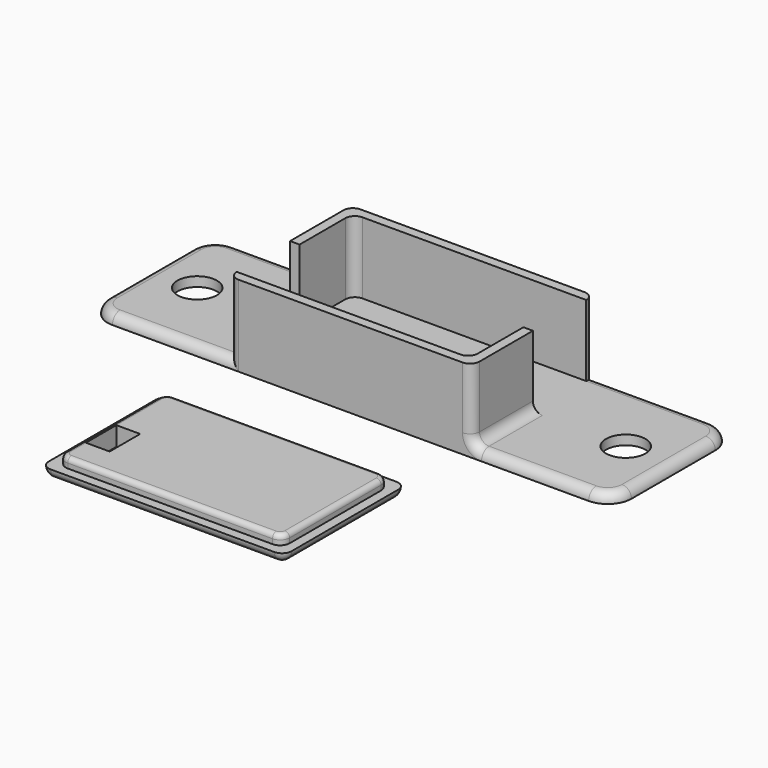
from build123d import *

# Parameters (mm, degrees)
F0_W      = 110
F0_H      = 32
F0_R      = 4.15
F1_DEPTH  = 2
F2_W      = 23.5
F2_H      = 2
F3_DEPTH  = 15
F4_W      = 14
F4_H      = 15
F5_DEPTH  = 2
F6_W      = 14
F6_H      = 15
F7_DEPTH  = 2
F8_R      = 5
F9_F1_R   = 2
F9_F2_R   = 1.9999
F10_W     = 51
F10_H     = 32
F10_W_2   = 47
F10_H_2   = 28
F11_DEPTH = 2
F12_W     = 23.5
F12_H     = 28
F13_DEPTH = 2
F14_R     = 1.99999
F15_R     = 1
F16_W     = 5
F16_H     = 8
F17_DEPTH = 25


# Not quite as in the source:
# - a fillet or chamfer is up to 0.001 mm smaller than in the source, because OpenCascade refuses the exact size


with BuildPart() as f1:
    # F0 (on Top) → F1 (new body)
    with BuildSketch(Plane.XY):
        Rectangle(F0_W, F0_H)
        with Locations((-45, 0)):
            Circle(F0_R, mode=Mode.SUBTRACT)
        with BuildLine():
            ThreePointArc((49.15, 0), (45, -4.15), (40.85, 0))
            ThreePointArc((40.85, 0), (45, 4.15), (49.15, 0))
        make_face(mode=Mode.SUBTRACT)
    extrude(amount=F1_DEPTH)

    # F2 (on face) → F3 (join)
    with BuildSketch(Plane.XY.offset(2)):
        with Locations((-11.75, -15)):
            Rectangle(F2_W, F2_H)
        with Locations((11.75, -15)):
            Rectangle(F2_W, F2_H)
        Polygon((23.5, -14), (23.5, -16), (25.5, -16), (25.5, 16), (23.5, 16), (23.5, 14), align=None)
        Polygon((-25.5, -16), (-23.5, -16), (-23.5, -14), (-23.5, 14), (-23.5, 16), (-25.5, 16), align=None)
        with Locations((-11.75, 15)):
            Rectangle(F2_W, F2_H)
        with Locations((11.75, 15)):
            Rectangle(F2_W, F2_H)
    extrude(amount=F3_DEPTH)

    # F4 (on face) → F5 (cut, through all)
    with BuildSketch(Plane(origin=(-25.5, 0, 0), x_dir=(0, -1, 0), z_dir=(-1, 0, 0))):
        with Locations((7, 9.5)):
            Rectangle(F4_W, F4_H)
    extrude(amount=-F5_DEPTH, mode=Mode.SUBTRACT)

    # F6 (on face) → F7 (cut, through all)
    with BuildSketch(Plane.YZ.offset(25.5)):
        with Locations((7, 9.5)):
            Rectangle(F6_W, F6_H)
    extrude(amount=-F7_DEPTH, mode=Mode.SUBTRACT)

    # F8
    f8_edges = [f1.edges().sort_by_distance(p)[0] for p in [
        (-55, -16, 1),
        (-55, 16, 1),
        (55, -16, 1),
        (55, 16, 1),
    ]]
    fillet(f8_edges, radius=F8_R)

    # F9: fillet of radius 2 on 8 edges, made by hand

    # F9_f1
    f9_f1_edges = [f1.edges().sort_by_distance(p)[0] for p in [
        (23.5, -14, 9.5),
        (-23.5, 14, 9.5),
        (-25.5, 8, 2),
        (25.5, -8, 2),
    ]]
    fillet(f9_f1_edges, radius=F9_F1_R)

    # F9_f2 (radius 2 in the source; OpenCascade refuses exactly that, so slightly less here)
    f9_f2_edges = [f1.edges().sort_by_distance(p)[0] for p in [
        (25.5, -16, 10.5),
        (-25.5, 16, 10.5),
        (25.5, 16, 9.5),
        (-25.5, -16, 9.5),
        (-26.0857864376, 16, 2.5857864376),
        (26.0857864376, -16, 2.5857864376),
    ]]
    fillet(f9_f2_edges, radius=F9_F2_R)


with BuildPart() as f11:
    # F10 (on Top) → F11 (new body)
    with BuildSketch(Plane.XY):
        with Locations((0, -49.3504135075)):
            Rectangle(F10_W, F10_H)
        with Locations((0, -49.3504135075)):
            Rectangle(F10_W_2, F10_H_2, mode=Mode.SUBTRACT)
        with Locations((0, -49.3504135075)):
            Rectangle(F10_W_2, F10_H_2)
    extrude(amount=F11_DEPTH)

    # F12 (on face) → F13 (join)
    with BuildSketch(Plane.XY.offset(2)):
        with Locations((11.75, -49.3504135075)):
            Rectangle(F12_W, F12_H)
        with Locations((-11.75, -49.3504135075)):
            Rectangle(F12_W, F12_H)
    extrude(amount=F13_DEPTH)

    # F14 (radius 2 in the source; OpenCascade refuses exactly that, so slightly less here)
    f14_edges = [f11.edges().sort_by_distance(p)[0] for p in [
        (-23.5, -63.350414, 3),
        (-25.5, -65.350414, 1),
        (23.5, -63.350414, 3),
        (23.5, -35.350414, 3),
        (-23.5, -35.350414, 3),
        (-25.5, -33.350414, 1),
        (25.5, -33.350414, 1),
        (25.5, -65.350414, 1),
        (0, -65.350414, 0),
        (25.5, -49.350414, 0),
        (0, -33.350414, 0),
        (-25.5, -49.350414, 0),
    ]]
    fillet(f14_edges, radius=F14_R)

    # F15
    f15_edges = [f11.edges().sort_by_distance(p)[0] for p in [
        (23.5, -49.350414, 4),
        (22.914216, -62.76463, 4),
        (22.914216, -35.936197, 4),
        (0, -63.350414, 4),
        (0, -35.350414, 4),
        (-22.914216, -62.76463, 4),
        (-22.914216, -35.936197, 4),
        (-23.5, -49.350414, 4),
    ]]
    fillet(f15_edges, radius=F15_R)

    # F16 (on face) → F17 (cut)
    with BuildSketch(Plane.XY.offset(4)):
        with Locations((-20, -53.3504135075)):
            Rectangle(F16_W, F16_H)
    extrude(amount=-F17_DEPTH, mode=Mode.SUBTRACT)


solid = Compound([f1.part, f11.part])
